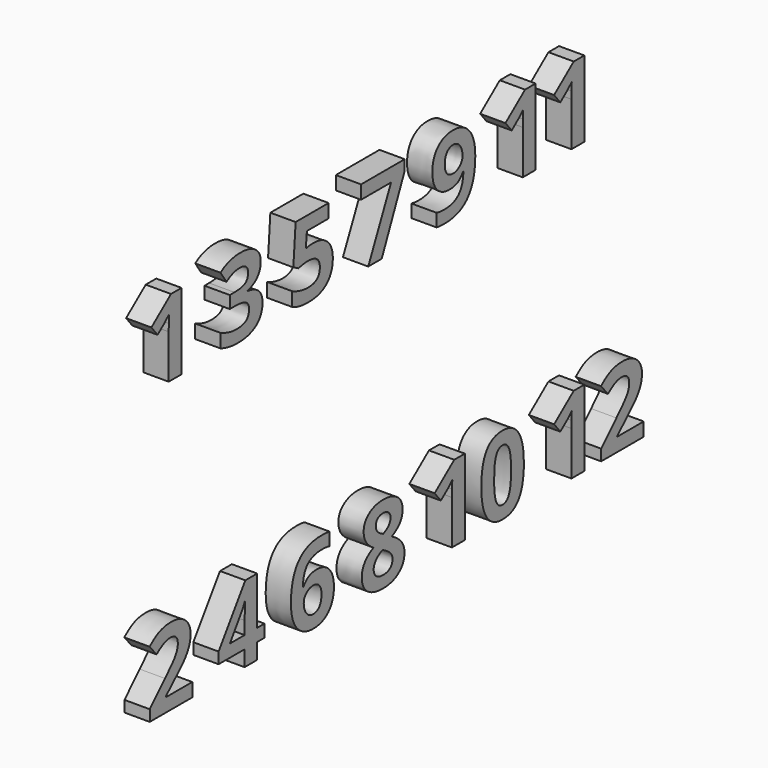
from build123d import *

# Parameters (mm, degrees)
F0_TEXT_SIZE = 12.6449853098
F1_DEPTH     = 3


# Not quite as in the source:
# - Text() gives the source's letters only with a copy of the font that has no kerning and outlines rounded to 1/6400 em; it was checked with that copy


with BuildPart() as f1:
    # F0 (on Right) → F1 (new body)
    with BuildSketch(Plane.YZ):
        with Locations((-74.5876313173, 0)):
            Text('1 3 5 7 9 11', F0_TEXT_SIZE, font='Open Sans', font_style=FontStyle.BOLD, text_align=(TextAlign.LEFT, TextAlign.BOTTOM))
        with Locations((-74.5876313173, -34.3943600427)):
            Text('2 4 6 8 10 12', F0_TEXT_SIZE, font='Open Sans', font_style=FontStyle.BOLD, text_align=(TextAlign.LEFT, TextAlign.BOTTOM))
    extrude(amount=F1_DEPTH)


solid = f1.part
